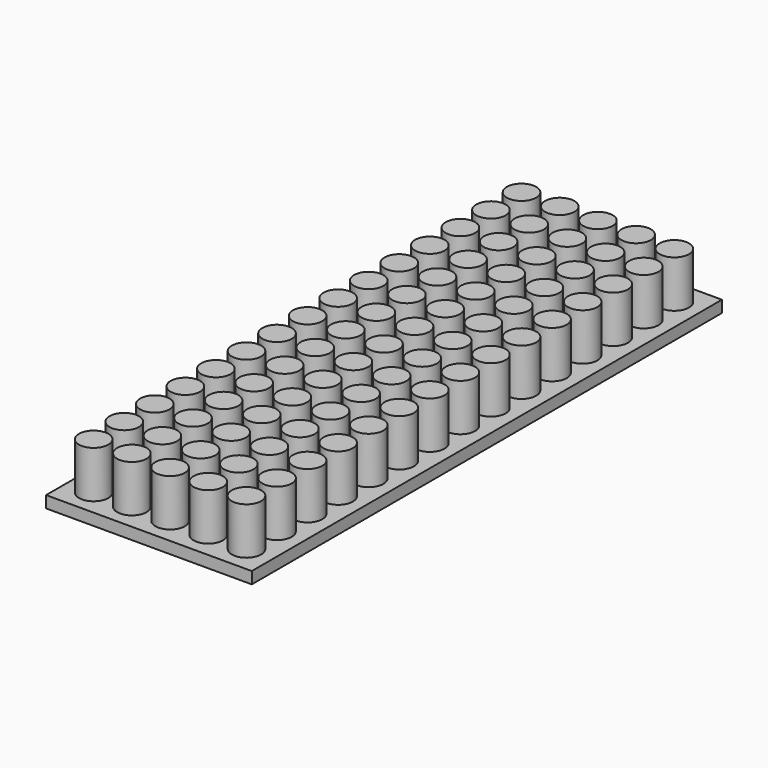
from build123d import *

# Parameters (mm, degrees)
F0_W     = 17.5
F0_H     = 50
F0_R     = 1.25
F1_DEPTH = 1
F2_DEPTH = 5


with BuildPart() as f1:
    # F0 (on Top) → F1 (new body)
    with BuildSketch(Plane.XY):
        Rectangle(F0_W, F0_H)
        with Locations((-6.5, -22.75)):
            Circle(F0_R, mode=Mode.SUBTRACT)
        with Locations((-6.5, -19.5)):
            Circle(F0_R, mode=Mode.SUBTRACT)
        with Locations((-6.5, -16.25)):
            Circle(F0_R, mode=Mode.SUBTRACT)
        with Locations((-6.5, -13)):
            Circle(F0_R, mode=Mode.SUBTRACT)
        with Locations((-3.25, -22.75)):
            Circle(F0_R, mode=Mode.SUBTRACT)
        with Locations((-3.25, -19.5)):
            Circle(F0_R, mode=Mode.SUBTRACT)
        with Locations((-3.25, -16.25)):
            Circle(F0_R, mode=Mode.SUBTRACT)
        with Locations((-3.25, -13)):
            Circle(F0_R, mode=Mode.SUBTRACT)
        with Locations((-6.5, -9.75)):
            Circle(F0_R, mode=Mode.SUBTRACT)
        with Locations((-6.5, -6.5)):
            Circle(F0_R, mode=Mode.SUBTRACT)
        with Locations((-6.5, -3.25)):
            Circle(F0_R, mode=Mode.SUBTRACT)
        with Locations((-3.25, -9.75)):
            Circle(F0_R, mode=Mode.SUBTRACT)
        with Locations((-3.25, -6.5)):
            Circle(F0_R, mode=Mode.SUBTRACT)
        with Locations((-3.25, -3.25)):
            Circle(F0_R, mode=Mode.SUBTRACT)
        with Locations((0, -22.75)):
            Circle(F0_R, mode=Mode.SUBTRACT)
        with Locations((0, -19.5)):
            Circle(F0_R, mode=Mode.SUBTRACT)
        with Locations((3.25, -22.75)):
            Circle(F0_R, mode=Mode.SUBTRACT)
        with Locations((3.25, -19.5)):
            Circle(F0_R, mode=Mode.SUBTRACT)
        with Locations((0, -16.25)):
            Circle(F0_R, mode=Mode.SUBTRACT)
        with Locations((0, -13)):
            Circle(F0_R, mode=Mode.SUBTRACT)
        with Locations((3.25, -16.25)):
            Circle(F0_R, mode=Mode.SUBTRACT)
        with Locations((3.25, -13)):
            Circle(F0_R, mode=Mode.SUBTRACT)
        with Locations((6.5, -22.75)):
            Circle(F0_R, mode=Mode.SUBTRACT)
        with Locations((6.5, -19.5)):
            Circle(F0_R, mode=Mode.SUBTRACT)
        with Locations((6.5, -16.25)):
            Circle(F0_R, mode=Mode.SUBTRACT)
        with Locations((6.5, -13)):
            Circle(F0_R, mode=Mode.SUBTRACT)
        with Locations((0, -9.75)):
            Circle(F0_R, mode=Mode.SUBTRACT)
        with Locations((0, -6.5)):
            Circle(F0_R, mode=Mode.SUBTRACT)
        with Locations((3.25, -9.75)):
            Circle(F0_R, mode=Mode.SUBTRACT)
        with Locations((3.25, -6.5)):
            Circle(F0_R, mode=Mode.SUBTRACT)
        with Locations((0, -3.25)):
            Circle(F0_R, mode=Mode.SUBTRACT)
        with Locations((3.25, -3.25)):
            Circle(F0_R, mode=Mode.SUBTRACT)
        with Locations((6.5, -9.75)):
            Circle(F0_R, mode=Mode.SUBTRACT)
        with Locations((6.5, -6.5)):
            Circle(F0_R, mode=Mode.SUBTRACT)
        with Locations((6.5, -3.25)):
            Circle(F0_R, mode=Mode.SUBTRACT)
        with Locations((-6.5, 0)):
            Circle(F0_R, mode=Mode.SUBTRACT)
        with Locations((-6.5, 3.25)):
            Circle(F0_R, mode=Mode.SUBTRACT)
        with Locations((-6.5, 6.5)):
            Circle(F0_R, mode=Mode.SUBTRACT)
        with Locations((-6.5, 9.75)):
            Circle(F0_R, mode=Mode.SUBTRACT)
        with Locations((-3.25, 0)):
            Circle(F0_R, mode=Mode.SUBTRACT)
        with Locations((-3.25, 3.25)):
            Circle(F0_R, mode=Mode.SUBTRACT)
        with Locations((-3.25, 6.5)):
            Circle(F0_R, mode=Mode.SUBTRACT)
        with Locations((-3.25, 9.75)):
            Circle(F0_R, mode=Mode.SUBTRACT)
        with Locations((-6.5, 13)):
            Circle(F0_R, mode=Mode.SUBTRACT)
        with Locations((-6.5, 16.25)):
            Circle(F0_R, mode=Mode.SUBTRACT)
        with Locations((-6.5, 19.5)):
            Circle(F0_R, mode=Mode.SUBTRACT)
        with Locations((-6.5, 22.75)):
            Circle(F0_R, mode=Mode.SUBTRACT)
        with Locations((-3.25, 13)):
            Circle(F0_R, mode=Mode.SUBTRACT)
        with Locations((-3.25, 16.25)):
            Circle(F0_R, mode=Mode.SUBTRACT)
        with Locations((-3.25, 19.5)):
            Circle(F0_R, mode=Mode.SUBTRACT)
        with Locations((-3.25, 22.75)):
            Circle(F0_R, mode=Mode.SUBTRACT)
        Circle(F0_R, mode=Mode.SUBTRACT)
        with Locations((0, 3.25)):
            Circle(F0_R, mode=Mode.SUBTRACT)
        with Locations((3.25, 0)):
            Circle(F0_R, mode=Mode.SUBTRACT)
        with Locations((3.25, 3.25)):
            Circle(F0_R, mode=Mode.SUBTRACT)
        with Locations((0, 6.5)):
            Circle(F0_R, mode=Mode.SUBTRACT)
        with Locations((0, 9.75)):
            Circle(F0_R, mode=Mode.SUBTRACT)
        with Locations((3.25, 6.5)):
            Circle(F0_R, mode=Mode.SUBTRACT)
        with Locations((3.25, 9.75)):
            Circle(F0_R, mode=Mode.SUBTRACT)
        with Locations((6.5, 0)):
            Circle(F0_R, mode=Mode.SUBTRACT)
        with Locations((6.5, 3.25)):
            Circle(F0_R, mode=Mode.SUBTRACT)
        with Locations((6.5, 6.5)):
            Circle(F0_R, mode=Mode.SUBTRACT)
        with Locations((6.5, 9.75)):
            Circle(F0_R, mode=Mode.SUBTRACT)
        with Locations((0, 13)):
            Circle(F0_R, mode=Mode.SUBTRACT)
        with Locations((0, 16.25)):
            Circle(F0_R, mode=Mode.SUBTRACT)
        with Locations((3.25, 13)):
            Circle(F0_R, mode=Mode.SUBTRACT)
        with Locations((3.25, 16.25)):
            Circle(F0_R, mode=Mode.SUBTRACT)
        with Locations((0, 19.5)):
            Circle(F0_R, mode=Mode.SUBTRACT)
        with Locations((0, 22.75)):
            Circle(F0_R, mode=Mode.SUBTRACT)
        with Locations((3.25, 19.5)):
            Circle(F0_R, mode=Mode.SUBTRACT)
        with Locations((3.25, 22.75)):
            Circle(F0_R, mode=Mode.SUBTRACT)
        with Locations((6.5, 13)):
            Circle(F0_R, mode=Mode.SUBTRACT)
        with Locations((6.5, 16.25)):
            Circle(F0_R, mode=Mode.SUBTRACT)
        with Locations((6.5, 19.5)):
            Circle(F0_R, mode=Mode.SUBTRACT)
        with Locations((6.5, 22.75)):
            Circle(F0_R, mode=Mode.SUBTRACT)
        with Locations((3.25, 0)):
            Circle(F0_R)
        with Locations((6.5, 0)):
            Circle(F0_R)
    extrude(amount=F1_DEPTH)

    # F0 (on Top) → F2 (join)
    with BuildSketch(Plane.XY):
        Circle(F0_R)
        with Locations((0, 3.25)):
            Circle(F0_R)
        with Locations((0, 6.5)):
            Circle(F0_R)
        with Locations((0, 9.75)):
            Circle(F0_R)
        with Locations((0, 13)):
            Circle(F0_R)
        with Locations((0, 16.25)):
            Circle(F0_R)
        with Locations((0, 19.5)):
            Circle(F0_R)
        with Locations((0, 22.75)):
            Circle(F0_R)
        with Locations((3.25, 0)):
            Circle(F0_R)
        with Locations((3.25, 3.25)):
            Circle(F0_R)
        with Locations((3.25, 6.5)):
            Circle(F0_R)
        with Locations((3.25, 9.75)):
            Circle(F0_R)
        with Locations((3.25, 13)):
            Circle(F0_R)
        with Locations((3.25, 16.25)):
            Circle(F0_R)
        with Locations((3.25, 19.5)):
            Circle(F0_R)
        with Locations((3.25, 22.75)):
            Circle(F0_R)
        with Locations((6.5, 0)):
            Circle(F0_R)
        with Locations((6.5, 3.25)):
            Circle(F0_R)
        with Locations((6.5, 6.5)):
            Circle(F0_R)
        with Locations((6.5, 9.75)):
            Circle(F0_R)
        with Locations((6.5, 13)):
            Circle(F0_R)
        with Locations((6.5, 16.25)):
            Circle(F0_R)
        with Locations((6.5, 19.5)):
            Circle(F0_R)
        with Locations((6.5, 22.75)):
            Circle(F0_R)
        with Locations((-3.25, 19.5)):
            Circle(F0_R)
        with Locations((-6.5, 9.75)):
            Circle(F0_R)
        with Locations((-6.5, 6.5)):
            Circle(F0_R)
        with Locations((-6.5, 16.25)):
            Circle(F0_R)
        with Locations((-6.5, 3.25)):
            Circle(F0_R)
        with Locations((-6.5, 22.75)):
            Circle(F0_R)
        with Locations((-6.5, 13)):
            Circle(F0_R)
        with Locations((-3.25, 13)):
            Circle(F0_R)
        with Locations((-3.25, 9.75)):
            Circle(F0_R)
        with Locations((-3.25, 6.5)):
            Circle(F0_R)
        with Locations((-3.25, 16.25)):
            Circle(F0_R)
        with Locations((-3.25, 3.25)):
            Circle(F0_R)
        with Locations((-3.25, 22.75)):
            Circle(F0_R)
        with Locations((-6.5, 19.5)):
            Circle(F0_R)
        with Locations((-3.25, -22.75)):
            Circle(F0_R)
        with Locations((-3.25, -19.5)):
            Circle(F0_R)
        with Locations((-3.25, -9.75)):
            Circle(F0_R)
        with Locations((-6.5, -16.25)):
            Circle(F0_R)
        with Locations((-3.25, -6.5)):
            Circle(F0_R)
        with Locations((-3.25, -16.25)):
            Circle(F0_R)
        with Locations((-3.25, -3.25)):
            Circle(F0_R)
        with Locations((-6.5, -9.75)):
            Circle(F0_R)
        with Locations((-6.5, -19.5)):
            Circle(F0_R)
        with Locations((-6.5, -22.75)):
            Circle(F0_R)
        with Locations((-6.5, -13)):
            Circle(F0_R)
        with Locations((-6.5, -6.5)):
            Circle(F0_R)
        with Locations((-6.5, -3.25)):
            Circle(F0_R)
        with Locations((-3.25, -13)):
            Circle(F0_R)
        with Locations((3.25, -13)):
            Circle(F0_R)
        with Locations((3.25, -9.75)):
            Circle(F0_R)
        with Locations((6.5, -16.25)):
            Circle(F0_R)
        with Locations((3.25, -6.5)):
            Circle(F0_R)
        with Locations((3.25, -3.25)):
            Circle(F0_R)
        with Locations((3.25, -22.75)):
            Circle(F0_R)
        with Locations((3.25, -19.5)):
            Circle(F0_R)
        with Locations((6.5, -6.5)):
            Circle(F0_R)
        with Locations((6.5, -19.5)):
            Circle(F0_R)
        with Locations((6.5, -13)):
            Circle(F0_R)
        with Locations((6.5, -3.25)):
            Circle(F0_R)
        with Locations((6.5, -22.75)):
            Circle(F0_R)
        with Locations((3.25, -16.25)):
            Circle(F0_R)
        with Locations((6.5, -9.75)):
            Circle(F0_R)
        with Locations((0, -6.5)):
            Circle(F0_R)
        with Locations((0, -9.75)):
            Circle(F0_R)
        with Locations((0, -22.75)):
            Circle(F0_R)
        with Locations((0, -19.5)):
            Circle(F0_R)
        with Locations((0, -16.25)):
            Circle(F0_R)
        with Locations((0, -13)):
            Circle(F0_R)
        with Locations((0, -3.25)):
            Circle(F0_R)
        with Locations((-6.5, 0)):
            Circle(F0_R)
        with Locations((-3.25, 0)):
            Circle(F0_R)
    extrude(amount=F2_DEPTH)


solid = f1.part
